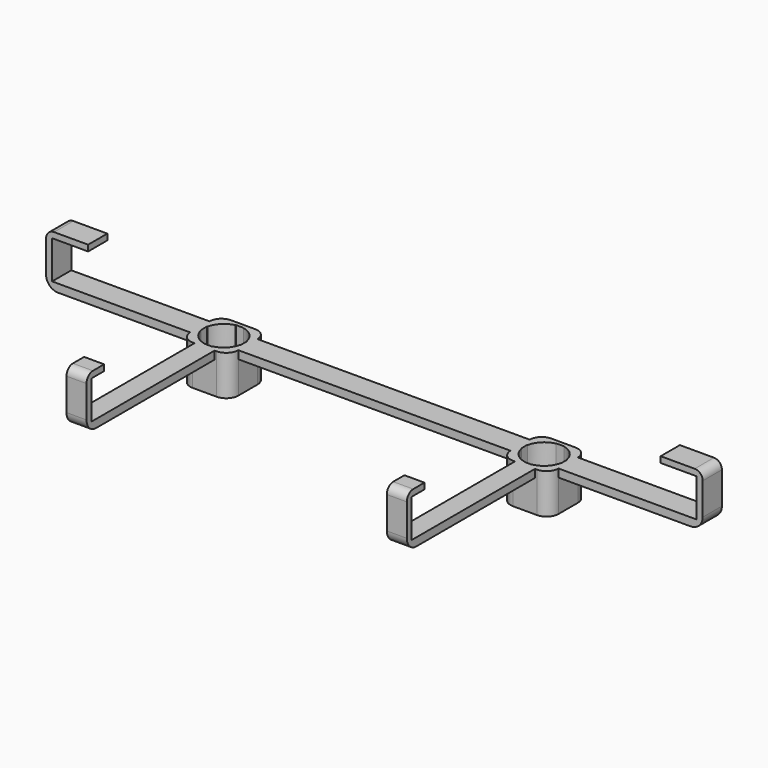
from build123d import *

# Parameters (mm, degrees)
F0_W      = 36
F0_H      = 6
F0_W_2    = 12
F0_H_2    = 3
F0_W_3    = 34
F0_W_4    = 2.5
F0_H_3    = 40
F1_DEPTH  = 2
F2_W      = 5
F2_H      = 1.5
F2_W_2    = 1.5
F2_H_2    = 6
F3_DEPTH  = 11
F4_W      = 5
F4_H      = 1.5
F5_DEPTH  = 4
F6_W      = 6
F6_H      = 1.5
F7_DEPTH  = 9
F8_W      = 6
F8_H      = 1.5
F9_DEPTH  = 9
F10_W     = 12
F10_H     = 12
F11_DEPTH = 8
F12_R     = 5
F13_DEPTH = 6
F15_DEPTH = 10
F16_R     = 2.99999
F17_R     = 2


# Not quite as in the source:
# - a fillet or chamfer is up to 0.001 mm smaller than in the source, because OpenCascade refuses the exact size


with BuildPart() as f1:
    # F0 (on Top) → F1 (new body)
    with BuildSketch(Plane.XY):
        with Locations((64, 0)):
            Rectangle(F0_W, F0_H)
        Polygon((46, -3), (46, 3), (34, 3), (34, 0), (34, -3), align=None)
        with Locations((40, 4.5)):
            Rectangle(F0_W_2, F0_H_2)
        Polygon((34, 0), (34, 3), (-34, 3), (-34, 0), (0, 0), align=None)
        Polygon((46, -6), (46, -3), (34, -3), (34, -6), (37.5, -6), (40, -6), (42.5, -6), align=None)
        Polygon((-34, 0), (-34, 3), (-46, 3), (-46, -3), (-34, -3), align=None)
        with Locations((-40, 4.5)):
            Rectangle(F0_W_2, F0_H_2)
        with Locations((17, -1.5)):
            Rectangle(F0_W_3, F0_H_2)
        with Locations((-64, 0)):
            Rectangle(F0_W, F0_H)
        with Locations((-17, -1.5)):
            Rectangle(F0_W_3, F0_H_2)
        with Locations((41.25, -26)):
            Rectangle(F0_W_4, F0_H_3)
        Polygon((-34, -3), (-46, -3), (-46, -6), (-42.5, -6), (-40, -6), (-37.5, -6), (-34, -6), align=None)
        with Locations((38.75, -26)):
            Rectangle(F0_W_4, F0_H_3)
        with Locations((-41.25, -26)):
            Rectangle(F0_W_4, F0_H_3)
        with Locations((-38.75, -26)):
            Rectangle(F0_W_4, F0_H_3)
    extrude(amount=F1_DEPTH)

    # F2 (on face) → F3 (join)
    with BuildSketch(Plane.XY.offset(2)):
        with Locations((-40, -45.25)):
            Rectangle(F2_W, F2_H)
        with Locations((40, -45.25)):
            Rectangle(F2_W, F2_H)
        with Locations((-81.25, 0)):
            Rectangle(F2_W_2, F2_H_2)
        with Locations((81.25, 0)):
            Rectangle(F2_W_2, F2_H_2)
    extrude(amount=F3_DEPTH)

    # F4 (on face) → F5 (join)
    with BuildSketch(Plane(origin=(0, -44.5, 0), x_dir=(-1, 0, 0), z_dir=(0, 1, 0))):
        with Locations((40, 12.25)):
            Rectangle(F4_W, F4_H)
        with Locations((-40, 12.25)):
            Rectangle(F4_W, F4_H)
    extrude(amount=F5_DEPTH)

    # F6 (on face) → F7 (join)
    with BuildSketch(Plane(origin=(80.5, 0, 0), x_dir=(0, -1, 0), z_dir=(-1, 0, 0))):
        with Locations((0, 12.25)):
            Rectangle(F6_W, F6_H)
    extrude(amount=F7_DEPTH)

    # F8 (on face) → F9 (join)
    with BuildSketch(Plane.YZ.offset(-80.5)):
        with Locations((0, 12.25)):
            Rectangle(F8_W, F8_H)
    extrude(amount=F9_DEPTH)

    # F10 (on face) → F11 (join)
    with BuildSketch(Plane(origin=(0, 0, 0), x_dir=(1, 0, 0), z_dir=(0, 0, -1))):
        with Locations((-40, 0)):
            Rectangle(F10_W, F10_H)
        with Locations((40, 0)):
            Rectangle(F10_W, F10_H)
    extrude(amount=F11_DEPTH)

    # F12 (on face) → F13 (cut)
    with BuildSketch(Plane.XY.offset(2)):
        with Locations((-40, 0)):
            Circle(F12_R)
        with Locations((40, 0)):
            Circle(F12_R)
    extrude(amount=-F13_DEPTH, mode=Mode.SUBTRACT)

    # F14 (on face) → F15 (cut)
    with BuildSketch(Plane(origin=(0, 0, -8), x_dir=(1, 0, 0), z_dir=(0, 0, -1))):
        with BuildLine():
            ThreePointArc((42.8284271247, -1), (42.956795679, -0.5073059362), (43, 0))
            ThreePointArc((43, 0), (42.956795679, 0.5073059362), (42.8284271247, 1))
            ThreePointArc((42.8284271247, 1), (42.1213203436, 2.1213203436), (41, 2.8284271247))
            ThreePointArc((41, 2.8284271247), (40, 3), (39, 2.8284271247))
            ThreePointArc((39, 2.8284271247), (37.8786796564, 2.1213203436), (37.1715728753, 1))
            ThreePointArc((37.1715728753, 1), (37, 0), (37.1715728753, -1))
            ThreePointArc((37.1715728753, -1), (37.8786796564, -2.1213203436), (39, -2.8284271247))
            ThreePointArc((39, -2.8284271247), (40, -3), (41, -2.8284271247))
            ThreePointArc((41, -2.8284271247), (42.1213203436, -2.1213203436), (42.8284271247, -1))
        make_face()
        with BuildLine():
            ThreePointArc((42.8284271247, 1), (42.956795679, 0.5073059362), (43, 0))
            ThreePointArc((43, 0), (42.956795679, -0.5073059362), (42.8284271247, -1))
            Line((42.8284271247, -1), (45, -1))
            Line((45, -1), (45, 0))
            Line((45, 0), (45, 1))
            Line((45, 1), (42.8284271247, 1))
        make_face()
        with BuildLine():
            ThreePointArc((39, 2.8284271247), (40, 3), (41, 2.8284271247))
            Line((41, 2.8284271247), (41, 5))
            Line((41, 5), (40, 5))
            Line((40, 5), (39, 5))
            Line((39, 5), (39, 2.8284271247))
        make_face()
        with BuildLine():
            Line((41, -5), (41, -2.8284271247))
            ThreePointArc((41, -2.8284271247), (40, -3), (39, -2.8284271247))
            Line((39, -2.8284271247), (39, -5))
            Line((39, -5), (40, -5))
            Line((40, -5), (41, -5))
        make_face()
        with BuildLine():
            ThreePointArc((37.1715728753, -1), (37, 0), (37.1715728753, 1))
            Line((37.1715728753, 1), (35, 1))
            Line((35, 1), (35, 0))
            Line((35, 0), (35, -1))
            Line((35, -1), (37.1715728753, -1))
        make_face()
        with BuildLine():
            ThreePointArc((-37.1715728753, -1), (-37.043204321, -0.5073059362), (-37, 0))
            ThreePointArc((-37, 0), (-37.043204321, 0.5073059362), (-37.1715728753, 1))
            ThreePointArc((-37.1715728753, 1), (-37.8786796564, 2.1213203436), (-39, 2.8284271247))
            ThreePointArc((-39, 2.8284271247), (-40, 3), (-41, 2.8284271247))
            ThreePointArc((-41, 2.8284271247), (-42.1213203436, 2.1213203436), (-42.8284271247, 1))
            ThreePointArc((-42.8284271247, 1), (-43, 0), (-42.8284271247, -1))
            ThreePointArc((-42.8284271247, -1), (-42.1213203436, -2.1213203436), (-41, -2.8284271247))
            ThreePointArc((-41, -2.8284271247), (-40, -3), (-39, -2.8284271247))
            ThreePointArc((-39, -2.8284271247), (-37.8786796564, -2.1213203436), (-37.1715728753, -1))
        make_face()
        with BuildLine():
            ThreePointArc((-37.1715728753, 1), (-37.043204321, 0.5073059362), (-37, 0))
            ThreePointArc((-37, 0), (-37.043204321, -0.5073059362), (-37.1715728753, -1))
            Line((-37.1715728753, -1), (-35, -1))
            Line((-35, -1), (-35, 0))
            Line((-35, 0), (-35, 1))
            Line((-35, 1), (-37.1715728753, 1))
        make_face()
        with BuildLine():
            ThreePointArc((-41, 2.8284271247), (-40, 3), (-39, 2.8284271247))
            Line((-39, 2.8284271247), (-39, 5))
            Line((-39, 5), (-40, 5))
            Line((-40, 5), (-41, 5))
            Line((-41, 5), (-41, 2.8284271247))
        make_face()
        with BuildLine():
            Line((-39, -5), (-39, -2.8284271247))
            ThreePointArc((-39, -2.8284271247), (-40, -3), (-41, -2.8284271247))
            Line((-41, -2.8284271247), (-41, -5))
            Line((-41, -5), (-40, -5))
            Line((-40, -5), (-39, -5))
        make_face()
        with BuildLine():
            ThreePointArc((-42.8284271247, -1), (-43, 0), (-42.8284271247, 1))
            Line((-42.8284271247, 1), (-45, 1))
            Line((-45, 1), (-45, 0))
            Line((-45, 0), (-45, -1))
            Line((-45, -1), (-42.8284271247, -1))
        make_face()
    extrude(amount=-F15_DEPTH, mode=Mode.SUBTRACT)

    # F16 (radius 3 in the source; OpenCascade refuses exactly that, so slightly less here)
    f16_edges = [f1.edges().sort_by_distance(p)[0] for p in [
        (-46, 6, -3),
        (-34, 6, -3),
        (-34, -6, -3),
        (-46, -6, -3),
        (46, 6, -3),
        (34, 6, -3),
        (46, -6, -3),
        (34, -6, -3),
        (40, -46, 0),
        (-40, -46, 0),
        (-82, 0, 0),
        (82, 0, 0),
    ]]
    fillet(f16_edges, radius=F16_R)

    # F17
    f17_edges = [f1.edges().sort_by_distance(p)[0] for p in [
        (-82, 0, 13),
        (-40, -46, 13),
        (40, -46, 13),
        (82, 0, 13),
    ]]
    fillet(f17_edges, radius=F17_R)


solid = f1.part
